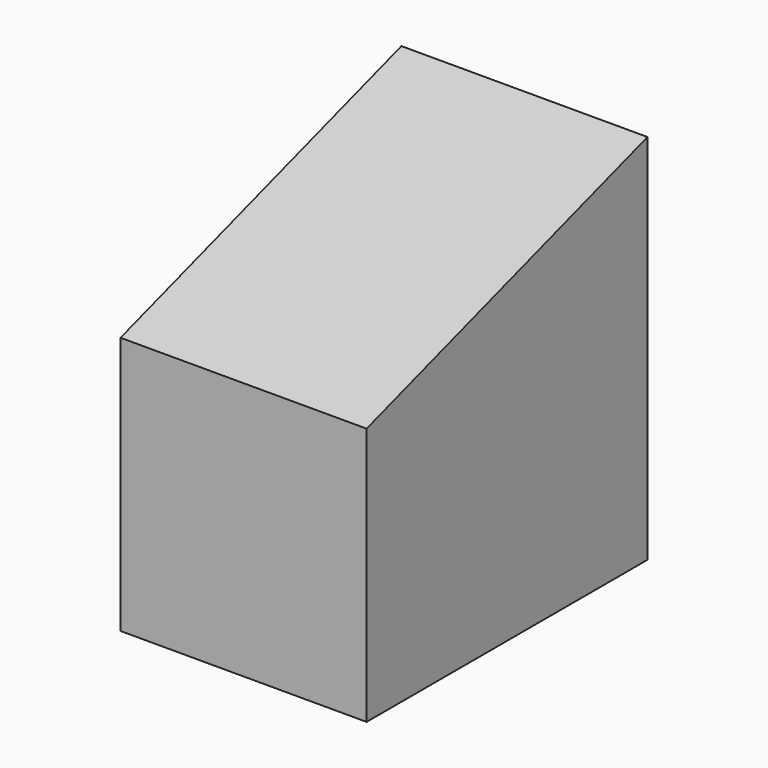
from build123d import *

# Parameters (mm, degrees)
F0_W     = 610
F0_H     = 640
F1_DEPTH = 870.217
F3_DEPTH = 610


# Not quite as in the source:
# - a feature names something its author has since deleted; it is built from what else it names


with BuildPart() as f1:
    # F0 (on Front) → F1 (new body)
    with BuildSketch(Plane.XZ):
        with Locations((-147.2222385816, -23.3099991456)):
            Rectangle(F0_W, F0_H)
    extrude(amount=F1_DEPTH)

    # F2 (on face) → F3 (join)
    with BuildSketch(Plane(origin=(-452.2222385816, 0, 0), x_dir=(0, -1, 0), z_dir=(-1, 0, 0))):
        Polygon((0, 296.6900008544), (870.217, 296.6900008544), (0, 579.4406441511), align=None)
    extrude(amount=-F3_DEPTH)


solid = f1.part
